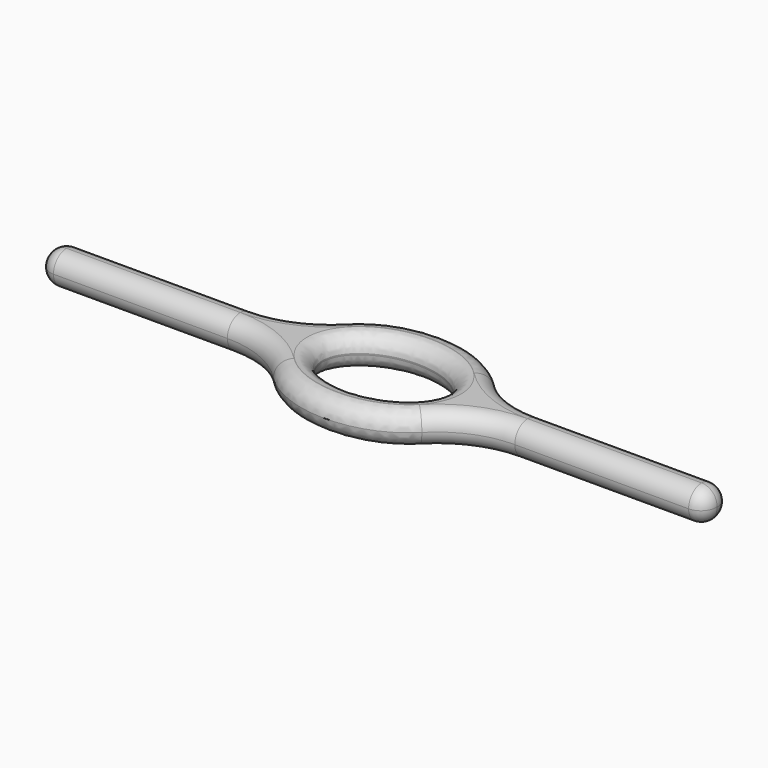
from build123d import *

# Parameters (mm, degrees)
F1_DEPTH = 3.175
F2_R     = 3.17499
F3_R     = 3.048
F4_R     = 3.048
F5_R     = 3.048


# Not quite as in the source:
# - a fillet or chamfer is up to 0.001 mm smaller than in the source, because OpenCascade refuses the exact size


with BuildPart() as f1:
    # F0 (on Top) → F1 (new body, symmetric)
    with BuildSketch(Plane.XY):
        with BuildLine():
            Line((65.3945878148, -3.175), (65.3945878148, 3.175))
            Line((65.3945878148, 3.175), (28.2152132282, 3.175))
            ThreePointArc((28.2152132282, 3.175), (20.8110387089, 4.67277223), (14.5711441877, 8.9305695865))
            add(Edge.make_bspline(
                [(14.5711441877, 8.9305695865), (0, 23.8849295035), (-14.5711441877, 8.9305695865)],
                knots=[0.657921386, 0.657921386, 0.657921386, 2.4836712676, 2.4836712676, 2.4836712676], degree=2, weights=[1, 0.6114734397, 1]))
            ThreePointArc((-14.5711441877, 8.9305695865), (-20.8110387089, 4.67277223), (-28.2152132282, 3.175))
            Line((-28.2152132282, 3.175), (-65.3945878148, 3.175))
            Line((-65.3945878148, 3.175), (-65.3945878148, -3.175))
            Line((-65.3945878148, -3.175), (-28.2152132282, -3.175))
            ThreePointArc((-28.2152132282, -3.175), (-20.8110387089, -4.67277223), (-14.5711441877, -8.9305695865))
            add(Edge.make_bspline(
                [(-14.5711441877, -8.9305695865), (0, -23.8849295035), (14.5711441877, -8.9305695865)],
                knots=[3.7995140395, 3.7995140395, 3.7995140395, 5.6252639212, 5.6252639212, 5.6252639212], degree=2, weights=[1, 0.6114734397, 1]))
            ThreePointArc((14.5711441877, -8.9305695865), (20.8110387089, -4.67277223), (28.2152132282, -3.175))
            Line((28.2152132282, -3.175), (65.3945878148, -3.175))
        make_face()
        with BuildLine():
            add(Edge.make_bspline(
                [(-12.065, 0), (-12.065, -14.2980794165), (6.0325, -7.1490397082), (24.13, 0), (6.0325, 7.1490397082), (-12.065, 14.2980794165), (-12.065, 0)],
                knots=[0, 0, 0, 2.0943951024, 2.0943951024, 4.1887902048, 4.1887902048, 6.2831853072, 6.2831853072, 6.2831853072], degree=2, weights=[1, 0.5, 1, 0.5, 1, 0.5, 1]))
        make_face(mode=Mode.SUBTRACT)
    extrude(amount=F1_DEPTH, both=True)

    # F2 (radius 3.175 in the source; OpenCascade refuses exactly that, so slightly less here)
    f2_edges = [f1.edges().sort_by_distance(p)[0] for p in [
        (-46.804901, -3.175, 3.175),
        (-46.804901, -3.175, -3.175),
        (-46.804901, 3.175, 3.175),
        (-46.804901, 3.175, -3.175),
        (20.811039, -4.672772, -3.175),
        (20.811039, -4.672772, 3.175),
        (0, -14.605, 3.175),
        (-20.811039, -4.672772, -3.175),
        (-20.811039, -4.672772, 3.175),
        (-20.811039, 4.672772, -3.175),
        (-20.811039, 4.672772, 3.175),
        (0, 14.605, 3.175),
        (20.811039, 4.672772, -3.175),
        (20.811039, 4.672772, 3.175),
        (46.804901, 3.175, -3.175),
        (46.804901, 3.175, 3.175),
        (0, 14.605, -3.175),
        (46.804901, -3.175, 3.175),
        (46.804901, -3.175, -3.175),
        (0, -14.605, -3.175),
    ]]
    fillet(f2_edges, radius=F2_R)

    # F3
    f3_edges = [f1.edges().sort_by_distance(p)[0] for p in [
        (65.394588, 2.245067, -2.245067),
    ]]
    fillet(f3_edges, radius=F3_R)

    # F4
    f4_edges = [f1.edges().sort_by_distance(p)[0] for p in [
        (-65.394588, 2.245067, -2.245067),
    ]]
    fillet(f4_edges, radius=F4_R)

    # F5
    f5_edges = [f1.edges().sort_by_distance(p)[0] for p in [
        (12.065, 0, 3.175),
        (12.065, 0, -3.175),
    ]]
    fillet(f5_edges, radius=F5_R)


solid = f1.part
